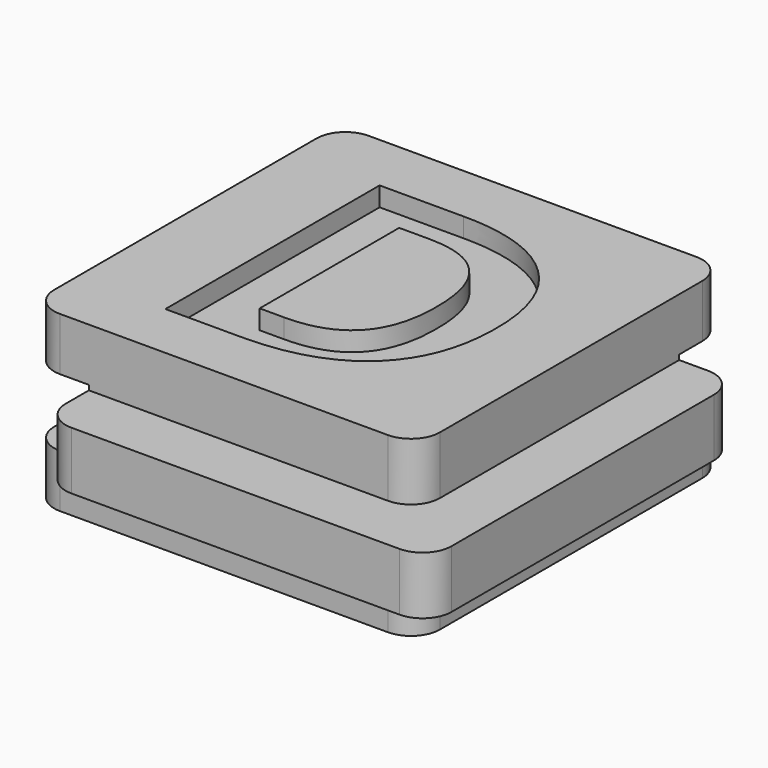
from build123d import *

# Parameters (mm, degrees)
F0_W         = 14
F0_H         = 3
F0_W_2       = 3
F1_DEPTH     = 20
F2_DEPTH     = 3
F3_W         = 3
F3_H         = 3
F4_DEPTH     = 100
F5_W         = 3
F5_H         = 3.5
F6_DEPTH     = 100
F7_R         = 1.5
F8_TEXT_SIZE = 19.4444444444
F9_DEPTH     = 1


# Not quite as in the source:
# - Text() gives the source's letters only with a copy of the font that has no kerning and outlines rounded to 1/6400 em; it was checked with that copy


with BuildPart() as f1:
    # F0 (on Front) → F1 (new body)
    with BuildSketch(Plane.XZ):
        Polygon((10, 1.5), (10, 4.5), (-10, 4.5), (-10, 1.5), (-7, 1.5), (7, 1.5), align=None)
        Rectangle(F0_W, F0_H)
        with Locations((11.5, 0)):
            Rectangle(F0_W_2, F0_H)
        with Locations((8.5, 0)):
            Rectangle(F0_W_2, F0_H)
        with Locations((-8.5, 0)):
            Rectangle(F0_W_2, F0_H)
        Polygon((10, -4.5), (10, -1.5), (7, -1.5), (-7, -1.5), (-10, -1.5), (-10, -4.5), align=None)
    extrude(amount=-F1_DEPTH)

    # F0 (on Front) → F2 (join)
    with BuildSketch(Plane.XZ):
        with Locations((-8.5, 0)):
            Rectangle(F0_W_2, F0_H)
        Rectangle(F0_W, F0_H)
        with Locations((8.5, 0)):
            Rectangle(F0_W_2, F0_H)
        with Locations((11.5, 0)):
            Rectangle(F0_W_2, F0_H)
    extrude(amount=F2_DEPTH)

    # F3 (on face) → F4 (cut)
    with BuildSketch(Plane.YZ.offset(13)):
        Polygon((23, -1.75), (23, 1.75), (17, 1.75), (17, 1.5), (20, 1.5), (20, -1.5), (17, -1.5), (17, -1.75), align=None)
        with Locations((18.5, 0)):
            Rectangle(F3_W, F3_H)
    extrude(amount=-F4_DEPTH, mode=Mode.SUBTRACT)

    # F5 (on face) → F6 (cut)
    with BuildSketch(Plane(origin=(0, 17, 0), x_dir=(-1, 0, 0), z_dir=(0, 1, 0))):
        with Locations((11.5, 0)):
            Rectangle(F5_W, F5_H)
        with Locations((8.5, 0)):
            Rectangle(F5_W, F5_H)
    extrude(amount=-F6_DEPTH, mode=Mode.SUBTRACT)

    # F7
    f7_edges = [f1.edges().sort_by_distance(p)[0] for p in [
        (-7, -3, 0),
        (13, -3, 0),
        (10, 0, 3),
        (10, 0, -3),
        (-10, 0, -3.125),
        (-10, 0, 3.125),
        (-7, 17, 0),
        (-10, 20, 3.125),
        (-10, 20, -3.125),
        (13, 17, 0),
        (10, 20, 3.125),
        (10, 20, -3.125),
    ]]
    fillet(f7_edges, radius=F7_R)

    # F8 (on face) → F9 (cut)
    with BuildSketch(Plane.XY.offset(4.5)):
        with Locations((-7.1801951318, 3)):
            Text('D', F8_TEXT_SIZE, font='Open Sans', font_style=FontStyle.BOLD, text_align=(TextAlign.LEFT, TextAlign.BOTTOM))
    extrude(amount=-F9_DEPTH, mode=Mode.SUBTRACT)


solid = f1.part
